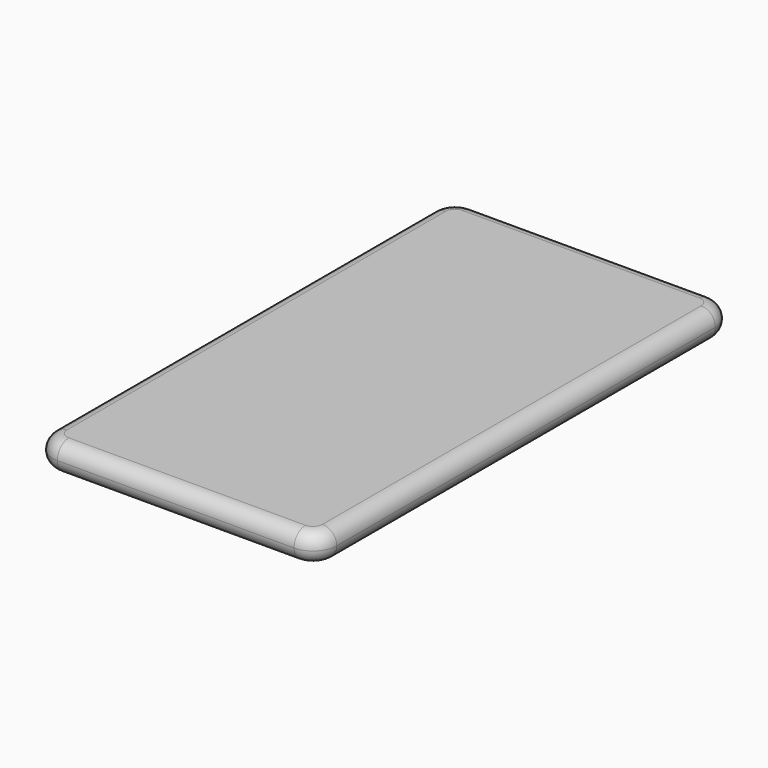
from build123d import *

# Parameters (mm, degrees)
F1_DEPTH = 7.62
F2_R     = 3.80999


# Not quite as in the source:
# - a fillet or chamfer is up to 0.001 mm smaller than in the source, because OpenCascade refuses the exact size


with BuildPart() as f1:
    # F0 (on Top) → F1 (new body)
    with BuildSketch(Plane.XY):
        with BuildLine():
            ThreePointArc((0, 6.35), (1.8598719395, 1.8598719395), (6.35, 0))
            Line((6.35, 0), (69.85, 0))
            ThreePointArc((69.85, 0), (74.3401280605, 1.8598719395), (76.2, 6.35))
            Line((76.2, 6.35), (76.2, 133.35))
            ThreePointArc((76.2, 133.35), (74.3401280605, 137.8401280605), (69.85, 139.7))
            Line((69.85, 139.7), (6.35, 139.7))
            ThreePointArc((6.35, 139.7), (1.8598719395, 137.8401280605), (0, 133.35))
            Line((0, 133.35), (0, 6.35))
        make_face()
    extrude(amount=F1_DEPTH)

    # F2 (radius 3.81 in the source; OpenCascade refuses exactly that, so slightly less here)
    f2_edges = [f1.edges().sort_by_distance(p)[0] for p in [
        (0, 69.85, 7.62),
        (0, 69.85, 0),
    ]]
    fillet(f2_edges, radius=F2_R)


solid = f1.part
